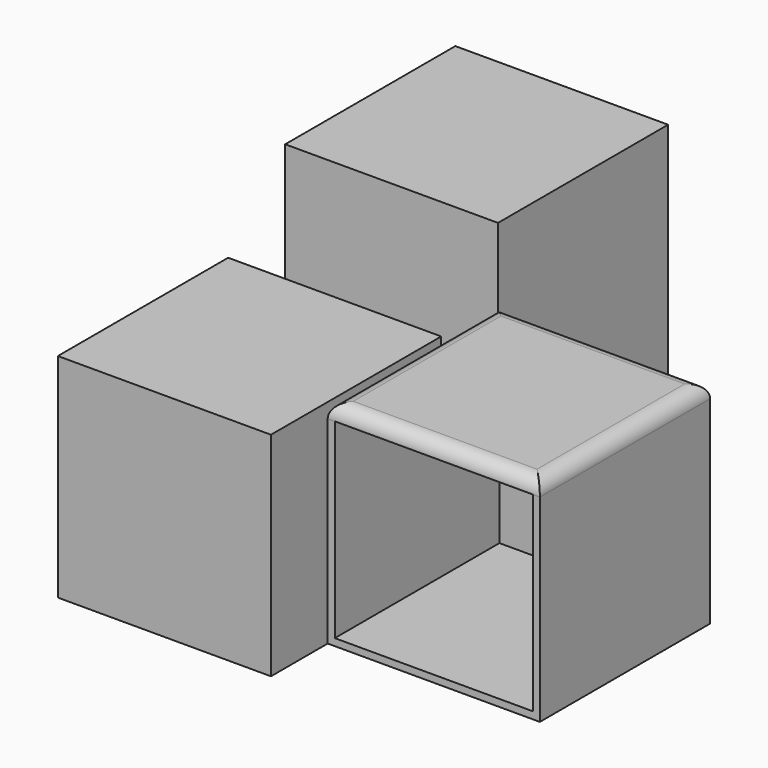
from build123d import *

# Parameters (mm, degrees)
F0_W     = 75.946
F0_H     = 75.9411230683
F1_DEPTH = 76.2
F3_R     = 5.08
F4_T     = -2.54
F5_W     = 76.2851387262
F5_H     = 76.1361420155
F6_DEPTH = 76.2
F7_W     = 76.178714633
F7_H     = 76.1255025864
F8_DEPTH = 101.6


# Not quite as in the source:
# - a shell that OpenCascade refuses in one call is made with other operations: the cavity is built on its own and cut out


with BuildPart() as f1:
    # F0 (on Front) → F1 (new body)
    with BuildSketch(Plane.XZ):
        with Locations((37.973, 37.9705615342)):
            Rectangle(F0_W, F0_H)
    extrude(amount=F1_DEPTH)

    # F3
    f3_edges = [f1.edges().sort_by_distance(p)[0] for p in [
        (75.946, -38.1, 75.941123),
        (0, -38.1, 75.941123),
        (37.973, 0, 75.941123),
        (37.973, -76.2, 75.941123),
    ]]
    fillet(f3_edges, radius=F3_R)

    # F4: a shell. OpenCascade refuses it in one call, so the cavity is built on its own and cut out:
    # the body offset inwards by the wall thickness, plus a prism from it out through each open face.
    f4_core = offset(f1.part, amount=F4_T, mode=Mode.PRIVATE)
    f4_exits = [f4_core.faces().sort_by_distance(p)[0] for p in [
        (37.973, -73.66, 36.700562),
    ]]
    add(f4_core, mode=Mode.SUBTRACT)
    extrude(f4_exits, amount=-F4_T, mode=Mode.SUBTRACT)

    # F5 (on offset) → F6 (join)
    with BuildSketch(Plane.XZ.offset(25.4)):
        with Locations((-38.1425693631, 38.0680710077)):
            Rectangle(F5_W, F5_H)
    extrude(amount=F6_DEPTH)


with BuildPart() as f8:
    # F7 (on Top) → F8 (new body)
    with BuildSketch(Plane.XY):
        with Locations((-38.0893573165, 38.0627512932)):
            Rectangle(F7_W, F7_H)
    extrude(amount=F8_DEPTH)


solid = Compound([f1.part, f8.part])
